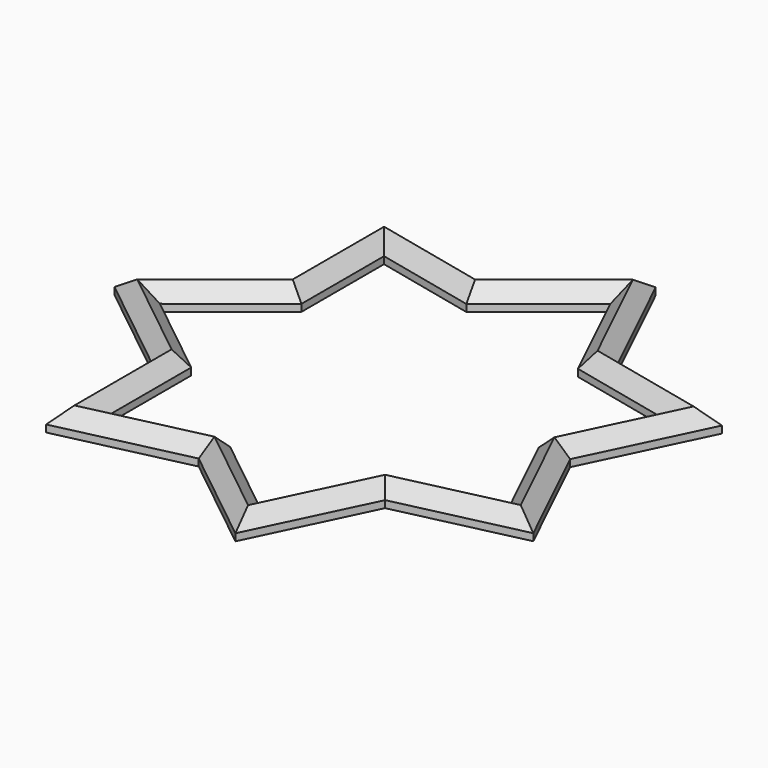
from build123d import *

# Parameters (mm, degrees)
F1_DEPTH = 3
F2_SIZE  = 1.99999


# Not quite as in the source:
# - a fillet or chamfer is up to 0.001 mm smaller than in the source, because OpenCascade refuses the exact size


with BuildPart() as f1:
    # F0 (on Top) → F1 (new body)
    with BuildSketch(Plane.XY):
        Polygon((6.0692586303, 20.150212978), (-2.1576516057, 37.2335681107), (-16.982031609, 25.4115195514), (-34.2207515071, 29.346144875), (-34.2207515071, 11.6640991742), (-48.8470692461, 0), (-34.2207515071, -11.6640991742), (-34.2207515071, -30.3718617382), (-15.982031609, -26.2089929403), (-1.6576516057, -37.6323048051), (6.2917795642, -21.1251408902), (24, -17.0833551327), (16.1191004999, -0.7184986964), (24.1784479339, 16.0169086929), align=None)
        Polygon((-42.4315673597, 0), (-30.2207515071, 9.737800699), (-30.2207515071, 24.3303035243), (-15.9941131941, 21.0831661669), (-3.5852350773, 30.9789162509), (3.3011727437, 16.6791430651), (18.3982804623, 13.2333267461), (11.6794354432, -0.7184986964), (18.2198325283, -14.2997731858), (3.5236936777, -17.6540709772), (-3.0852350773, -31.3776529454), (-14.9941131941, -21.8806395557), (-30.2207515071, -25.3560203876), (-30.2207515071, -9.737800699), align=None, mode=Mode.SUBTRACT)
    extrude(amount=F1_DEPTH)

    # F2 (size 2 in the source; OpenCascade refuses exactly that, so slightly less here)
    f2_edges = [f1.edges().sort_by_distance(p)[0] for p in [
        (15.123853, 18.083561, 3),
        (1.955804, 28.691891, 3),
        (-9.569842, 31.322544, 3),
        (-25.601392, 27.378832, 3),
        (-34.220752, 20.505122, 3),
        (-41.53391, 5.83205, 3),
        (-41.53391, -5.83205, 3),
        (-34.220752, -21.01798, 3),
        (-25.101392, -28.290427, 3),
        (-8.819842, -31.920649, 3),
        (2.317064, -29.378723, 3),
        (15.14589, -19.104248, 3),
        (20.05955, -8.900927, 3),
        (20.148774, 7.649205, 3),
        (-9.039674, -26.629146, 3),
        (-22.607432, -23.61833, 3),
        (-30.220752, -17.546911, 3),
        (-36.326159, -4.8689, 3),
        (-36.326159, 4.8689, 3),
        (-30.220752, 17.034052, 3),
        (-23.107432, 22.706735, 3),
        (-9.789674, 26.031041, 3),
        (-0.142031, 23.82903, 3),
        (10.849727, 14.956235, 3),
        (15.038858, 6.257414, 3),
        (14.949634, -7.509136, 3),
        (10.871763, -15.976922, 3),
        (0.219229, -24.515862, 3),
    ]]
    chamfer(f2_edges, length=F2_SIZE)


solid = f1.part
